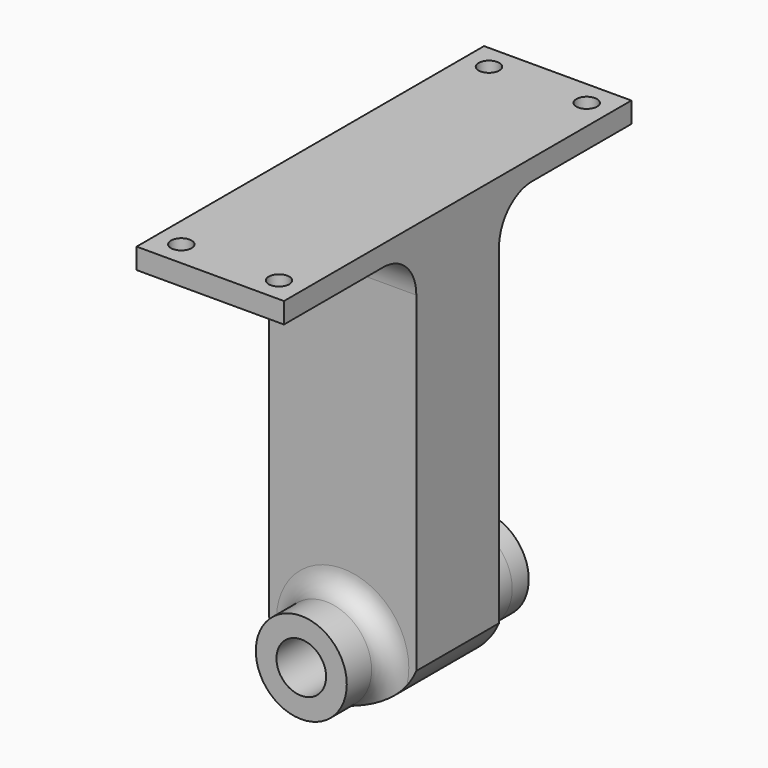
from build123d import *

# Parameters (mm, degrees)
F0_R         = 11
F0_R_2       = 6
F1_DEPTH     = 25
F2_R         = 11
F3_DEPTH     = 5
F5_DEPTH     = 12.5
F7_DEPTH     = 5
F8_R         = 10
F9_T4_ANGLE  = 90
F9_S5_R      = 18.3546430422
F9_T6_DEPTH  = 14
F9_T10_ANGLE = 270
F9_S11_R     = 18.3546430422
F9_T12_DEPTH = 26
F9_T16_ANGLE = 270
F9_S17_R     = 18.3546430422
F9_T18_DEPTH = 26
F9_T22_ANGLE = 270
F9_S23_R     = 18.3546430422
F9_T24_DEPTH = 26
F9_T28_ANGLE = 270
F9_S29_R     = 18.3546430422
F9_T30_DEPTH = 26
F9_T34_ANGLE = 90
F9_S35_R     = 18.3546430422
F9_T36_DEPTH = 14
F10_R        = 6
F11_DEPTH    = 30
F12_R        = 2.5
F13_DEPTH    = 5.001


# Not quite as in the source:
# - a fillet or chamfer that OpenCascade refuses, or shapes differently, is made with other operations: its cross-section is extruded or revolved along the edge and cut away or added


with BuildPart() as f1:
    # F0 (on Front) → F1 (new body, symmetric)
    with BuildSketch(Plane.XZ):
        Circle(F0_R)
        Circle(F0_R_2, mode=Mode.SUBTRACT)
    extrude(amount=F1_DEPTH, both=True)

    # F2 (on face) → F3 (join)
    with BuildSketch(Plane(origin=(0, 25, 0), x_dir=(-1, 0, 0), z_dir=(0, 1, 0))):
        Circle(F2_R)
    extrude(amount=F3_DEPTH)

    # F4 (on Front) → F5 (join, symmetric)
    with BuildSketch(Plane.XZ):
        with BuildLine():
            ThreePointArc((-17.8147200495, 0), (-10.6296195649, -8.2892337781), (0, -11))
            ThreePointArc((0, -11), (10.6296195649, -8.2892337781), (17.8147200495, 0))
            Line((17.8147200495, 0), (17.8147200495, 90))
            Line((17.8147200495, 90), (-17.8147200495, 90))
            Line((-17.8147200495, 90), (-17.8147200495, 0))
        make_face()
        with BuildLine():
            ThreePointArc((0, -11), (-7.7781745931, 7.7781745931), (11, 0))
            ThreePointArc((11, 0), (7.7781745931, -7.7781745931), (0, -11))
        make_face(mode=Mode.SUBTRACT)
        with BuildLine():
            ThreePointArc((0, -11), (7.7781745931, -7.7781745931), (11, 0))
            ThreePointArc((11, 0), (-7.7781745931, 7.7781745931), (0, -11))
        make_face()
    extrude(amount=F5_DEPTH, both=True)

    # F6 (on face) → F7 (join)
    with BuildSketch(Plane.XY.offset(90)):
        Polygon((17.8147200495, -52.5), (17.8147200495, -12.5), (17.8147200495, 12.5), (17.8147200495, 52.5), (-17.8147200495, 52.5), (-17.8147200495, 12.5), (-17.8147200495, -12.5), (-17.8147200495, -52.5), align=None)
    extrude(amount=F7_DEPTH)

    # F8
    f8_edges = [f1.edges().sort_by_distance(p)[0] for p in [
        (0, -12.5, 90),
        (0, 12.5, 90),
    ]]
    fillet(f8_edges, radius=F8_R)

    # F9: fillet of radius 5 on 4 edges, made by hand


with BuildPart() as f9_tool2:
    # F9_s3 → F9_t4 (revolve)
    with BuildSketch(Plane.YZ):
        with BuildLine():
            ThreePointArc((-12.5, -16), (-13.9644660941, -12.4644660941), (-17.5, -11))
            Line((-17.5, -11), (-12.5, -11))
            Line((-12.5, -11), (-12.5, -16))
        make_face()
    revolve(axis=Axis((0, -12.5, 0), (0, -1, 0)), revolution_arc=F9_T4_ANGLE)

    # F9_s5 → F9_t6 (intersect, symmetric)
    with BuildSketch(Plane.XZ.offset(16.8)):
        with Locations((0.9864220241, 7.3281175465)):
            Circle(F9_S5_R)
    extrude(amount=F9_T6_DEPTH, both=True, mode=Mode.INTERSECT)


with BuildPart() as f1_1:
    add(f1.part)

    # F9_t1: union F9_tool2
    add(f9_tool2.part)


with BuildPart() as f9_tool8:
    # F9_s9 → F9_t10 (revolve)
    with BuildSketch(Plane.XY):
        with BuildLine():
            ThreePointArc((16, -12.5), (12.4644660941, -13.9644660941), (11, -17.5))
            Line((11, -17.5), (11, -12.5))
            Line((11, -12.5), (16, -12.5))
        make_face()
    revolve(axis=Axis((0, -12.5, 0), (0, -1, 0)), revolution_arc=F9_T10_ANGLE)

    # F9_s11 → F9_t12 (intersect, symmetric)
    with BuildSketch(Plane.XZ.offset(16.8)):
        with Locations((0.9864220241, 7.3281175465)):
            Circle(F9_S11_R)
    extrude(amount=F9_T12_DEPTH, both=True, mode=Mode.INTERSECT)


with BuildPart() as f1_2:
    add(f1_1.part)

    # F9_t7: union F9_tool8
    add(f9_tool8.part)


with BuildPart() as f9_tool14:
    # F9_s15 → F9_t16 (revolve)
    with BuildSketch(Plane.XY):
        with BuildLine():
            ThreePointArc((16, -12.5), (12.4644660941, -13.9644660941), (11, -17.5))
            Line((11, -17.5), (11, -12.5))
            Line((11, -12.5), (16, -12.5))
        make_face()
    revolve(axis=Axis((0, -12.5, 0), (0, -1, 0)), revolution_arc=F9_T16_ANGLE)

    # F9_s17 → F9_t18 (intersect, symmetric)
    with BuildSketch(Plane.XZ.offset(16.8)):
        with Locations((-0.9864220241, 7.3281175465)):
            Circle(F9_S17_R)
    extrude(amount=F9_T18_DEPTH, both=True, mode=Mode.INTERSECT)


with BuildPart() as f1_3:
    add(f1_2.part)

    # F9_t13: union F9_tool14
    add(f9_tool14.part)


with BuildPart() as f9_tool20:
    # F9_s21 → F9_t22 (revolve)
    with BuildSketch(Plane.XY):
        with BuildLine():
            ThreePointArc((16, 12.5), (12.4644660941, 13.9644660941), (11, 17.5))
            Line((11, 17.5), (11, 12.5))
            Line((11, 12.5), (16, 12.5))
        make_face()
    revolve(axis=Axis((0, 12.5, 0), (0, -1, 0)), revolution_arc=F9_T22_ANGLE)

    # F9_s23 → F9_t24 (intersect, symmetric)
    with BuildSketch(Plane.XZ.offset(-16.8)):
        with Locations((0.9864220241, 7.3281175465)):
            Circle(F9_S23_R)
    extrude(amount=F9_T24_DEPTH, both=True, mode=Mode.INTERSECT)


with BuildPart() as f1_4:
    add(f1_3.part)

    # F9_t19: union F9_tool20
    add(f9_tool20.part)


with BuildPart() as f9_tool26:
    # F9_s27 → F9_t28 (revolve)
    with BuildSketch(Plane.XY):
        with BuildLine():
            ThreePointArc((16, 12.5), (12.4644660941, 13.9644660941), (11, 17.5))
            Line((11, 17.5), (11, 12.5))
            Line((11, 12.5), (16, 12.5))
        make_face()
    revolve(axis=Axis((0, 12.5, 0), (0, -1, 0)), revolution_arc=F9_T28_ANGLE)

    # F9_s29 → F9_t30 (intersect, symmetric)
    with BuildSketch(Plane.XZ.offset(-16.8)):
        with Locations((-0.9864220241, 7.3281175465)):
            Circle(F9_S29_R)
    extrude(amount=F9_T30_DEPTH, both=True, mode=Mode.INTERSECT)


with BuildPart() as f1_5:
    add(f1_4.part)

    # F9_t25: union F9_tool26
    add(f9_tool26.part)


with BuildPart() as f9_tool32:
    # F9_s33 → F9_t34 (revolve)
    with BuildSketch(Plane.YZ):
        with BuildLine():
            ThreePointArc((12.5, -16), (13.9644660941, -12.4644660941), (17.5, -11))
            Line((17.5, -11), (12.5, -11))
            Line((12.5, -11), (12.5, -16))
        make_face()
    revolve(axis=Axis((0, 12.5, 0), (0, -1, 0)), revolution_arc=F9_T34_ANGLE)

    # F9_s35 → F9_t36 (intersect, symmetric)
    with BuildSketch(Plane.XZ.offset(-16.8)):
        with Locations((0.9864220241, 7.3281175465)):
            Circle(F9_S35_R)
    extrude(amount=F9_T36_DEPTH, both=True, mode=Mode.INTERSECT)


with BuildPart() as f1_6:
    add(f1_5.part)

    # F9_t31: union F9_tool32
    add(f9_tool32.part)

    # F10 (on face) → F11 (cut)
    with BuildSketch(Plane.XZ.offset(12.5)):
        Circle(F10_R)
    extrude(amount=-F11_DEPTH, mode=Mode.SUBTRACT)

    # F12 (on face) → F13 (cut, through all)
    with BuildSketch(Plane(origin=(0, 0, 90), x_dir=(1, 0, 0), z_dir=(0, 0, -1))):
        with Locations((-11.8147200495, 46.5)):
            Circle(F12_R)
        with Locations((11.8147200495, 46.5)):
            Circle(F12_R)
        with Locations((-11.8147200495, -46.5)):
            Circle(F12_R)
        with Locations((11.8147200495, -46.5)):
            Circle(F12_R)
    extrude(amount=-F13_DEPTH, mode=Mode.SUBTRACT)


solid = f1_6.part
